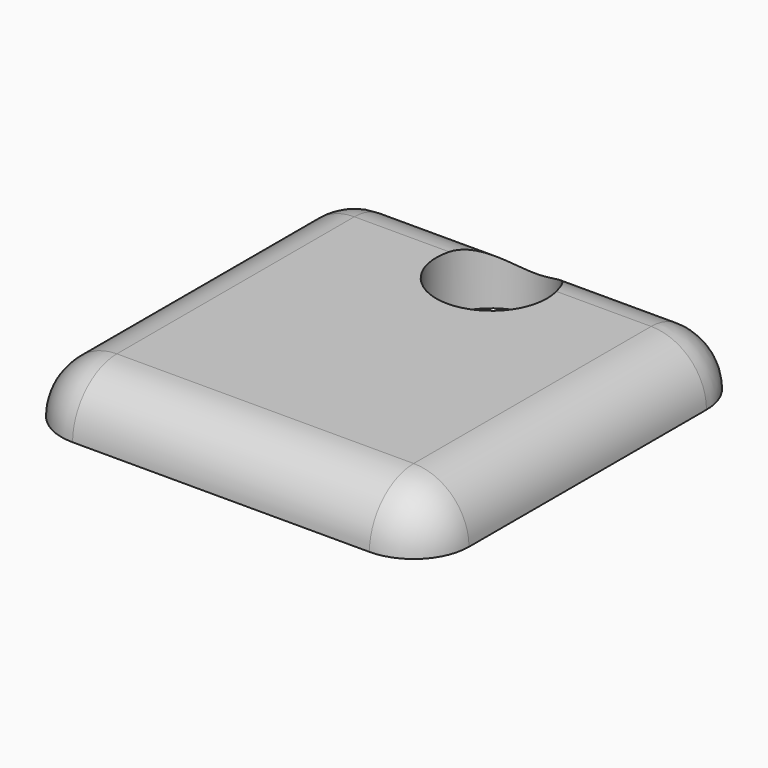
from build123d import *

# Parameters (mm, degrees)
F0_W        = 37.4135075825
F0_H        = 37.4135057104
F0_R        = 5.08
F1_DEPTH    = 5.08
F2_R        = 5.07999
F3_R        = 5.07999
F4_T1_DEPTH = 57.7335175825
F4_T3_DEPTH = 25.40001
F4_T6_ANGLE = 90
F5_R        = 5.07999


# Not quite as in the source:
# - a fillet or chamfer that OpenCascade refuses, or shapes differently, is made with other operations: its cross-section is extruded or revolved along the edge and cut away or added
# - a fillet or chamfer is up to 0.001 mm smaller than in the source, because OpenCascade refuses the exact size


with BuildPart() as f1:
    # F0 (on Top) → F1 (new body)
    with BuildSketch(Plane.XY):
        with Locations((-26.0004317388, 35.8758829534)):
            Rectangle(F0_W, F0_H)
        with Locations((-26.0004317388, 48.2149645656)):
            Circle(F0_R, mode=Mode.SUBTRACT)
    extrude(amount=F1_DEPTH)

    # F2 (radius 5.08 in the source; OpenCascade refuses exactly that, so slightly less here)
    f2_edges = [f1.edges().sort_by_distance(p)[0] for p in [
        (-26.000432, 17.16913, 5.08),
    ]]
    fillet(f2_edges, radius=F2_R)

    # F3 (radius 5.08 in the source; OpenCascade refuses exactly that, so slightly less here)
    f3_edges = [f1.edges().sort_by_distance(p)[0] for p in [
        (-7.293678, 38.415878, 5.08),
    ]]
    fillet(f3_edges, radius=F3_R)

    # F4: fillet of radius 5.08 on 1 edges, made by hand

    # F4_s2 → F4_t1 (cut)
    with BuildSketch(Plane.YZ.offset(-57.40718553)):
        with BuildLine():
            ThreePointArc((54.5826358086, 0), (53.094738257, 3.5921024484), (49.5026358086, 5.08))
            Line((49.5026358086, 5.08), (54.5826358086, 5.08))
            Line((54.5826358086, 5.08), (54.5826358086, 0))
        make_face()
    extrude(amount=F4_T1_DEPTH, mode=Mode.SUBTRACT)

    # F4_s4 → F4_t3 (cut)
    with BuildSketch(Plane.XY.offset(-12.7)):
        with BuildLine():
            ThreePointArc((-7.2936779475, 49.5026358086), (-8.7815754991, 53.094738257), (-12.3736779475, 54.5826358086))
            Line((-12.3736779475, 54.5826358086), (-7.2936779475, 54.5826358086))
            Line((-7.2936779475, 54.5826358086), (-7.2936779475, 49.5026358086))
        make_face()
    extrude(amount=F4_T3_DEPTH, mode=Mode.SUBTRACT)

    # F4_s5 → F4_t6 (revolve, cut)
    with BuildSketch(Plane.XY.offset(1e-05)):
        with BuildLine():
            ThreePointArc((-12.3736679475, 54.5826358086), (-8.7815719636, 53.0947347215), (-7.2936779475, 49.5026358086))
            Line((-7.2936779475, 49.5026358086), (-7.2936779475, 54.5826358086))
            Line((-7.2936779475, 54.5826358086), (-12.3736679475, 54.5826358086))
        make_face()
    revolve(axis=Axis((-12.3736679475, 54.5826358086, 1e-05), (0, -1, 0)), revolution_arc=F4_T6_ANGLE, mode=Mode.SUBTRACT)

    # F5 (radius 5.08 in the source; OpenCascade refuses exactly that, so slightly less here)
    f5_edges = [f1.edges().sort_by_distance(p)[0] for p in [
        (-44.707186, 35.875878, 5.08),
        (-44.707186, 17.16913, 5e-06),
        (-44.707186, 18.657025, 3.592105),
        (-44.707186, 53.094738, 3.592102),
    ]]
    fillet(f5_edges, radius=F5_R)


solid = f1.part
